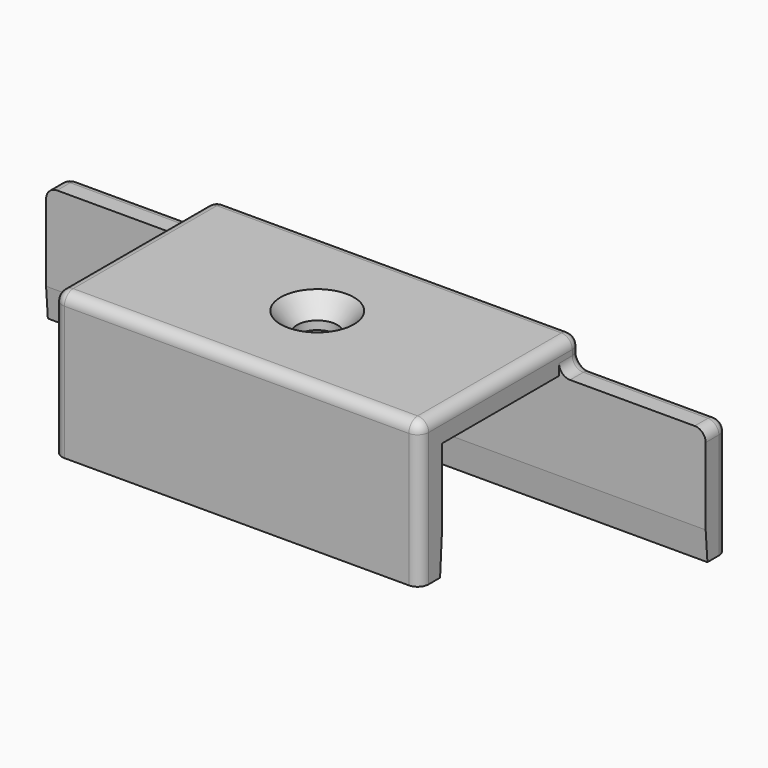
from build123d import *

# Parameters (mm, degrees)
F1_DEPTH       = 31.75
F4_D           = 6.985
F4_DEPTH       = 12.7
F4_CSINK_D     = 12.7
F4_CSINK_ANGLE = 82
F4_TIP         = 2.098505712
F5_SIZE2       = 0.381
F5_SIZE        = 6.35
F2_W           = 4.7625
F2_H           = 20.32
F6_DEPTH       = 25.4
F7_SIZE2       = 5.08
F7_SIZE        = 0.381
F8_R           = 1.905
F9_T1_DEPTH    = 23.1775
F9_T3_DEPTH    = 27.94
F9_S7_W        = 1.905
F9_S7_H        = 1.905
F9_T8_DEPTH    = 1.905
F9_S13_W       = 1.905
F9_S13_H       = 1.905
F9_T14_DEPTH   = 1.905
F9_S19_W       = 1.905
F9_S19_H       = 1.905
F9_T20_DEPTH   = 1.905
F9_S25_W       = 1.905
F9_S25_H       = 1.905
F9_T26_DEPTH   = 1.905


# Not quite as in the source:
# - a fillet or chamfer that OpenCascade refuses, or shapes differently, is made with other operations: its cross-section is extruded or revolved along the edge and cut away or added


with BuildPart() as f1:
    # F0 (on Right) → F1 (new body, symmetric)
    with BuildSketch(Plane.YZ):
        Polygon((-12.7, 0), (-12.7, 20.32), (12.7, 20.32), (12.7, 0), (17.4625, 0), (17.4625, 25.0825), (-17.4625, 25.0825), (-17.4625, 0), align=None)
    extrude(amount=F1_DEPTH, both=True)

    # F4
    with Locations(Plane.XY.offset(25.0825)):
        with Locations((0, 0)):
            CounterSinkHole(F4_D / 2, F4_CSINK_D / 2, depth=F4_DEPTH, counter_sink_angle=F4_CSINK_ANGLE)
            with Locations((0, 0, -(F4_DEPTH + F4_TIP / 2))):  # 118° drill point
                Cone(0, F4_D / 2, F4_TIP, mode=Mode.SUBTRACT)

    # F5
    f5_edges = [f1.edges().sort_by_distance(p)[0] for p in [
        (0, -12.7, 0),
    ]]
    f5_side = f1.faces().sort_by_distance((0, -12.7, 10.16))[0]
    chamfer(f5_edges, length=F5_SIZE, length2=F5_SIZE2, reference=f5_side)

    # F2 (on face) → F6 (join)
    with BuildSketch(Plane(origin=(-31.75, 0, 0), x_dir=(0, -1, 0), z_dir=(-1, 0, 0))):
        with Locations((-15.08125, 10.16)):
            Rectangle(F2_W, F2_H)
    extrude(amount=F6_DEPTH)

    # F7
    f7_edges = [f1.edges().sort_by_distance(p)[0] for p in [
        (-12.7, 12.7, 0),
    ]]
    chamfer(f7_edges, length=F7_SIZE, length2=F7_SIZE2)

    # F8
    f8_edges = [f1.edges().sort_by_distance(p)[0] for p in [
        (-31.75, 0, 25.0825),
        (-31.75, 15.08125, 20.32),
        (-57.15, 15.08125, 20.32),
        (31.75, 0, 25.0825),
        (0, 17.4625, 25.0825),
        (-31.75, 17.4625, 22.70125),
        (-44.45, 17.4625, 20.32),
        (0, -17.4625, 25.0825),
    ]]
    fillet(f8_edges, radius=F8_R)

    # F9: fillet of radius 1.905 on 4 edges, made by hand

    # F9_s2 → F9_t1 (cut)
    with BuildSketch(Plane.XY.offset(-4.7625)):
        with BuildLine():
            ThreePointArc((-55.245, 17.4625), (-56.5920384182, 16.9045384182), (-57.15, 15.5575))
            Line((-57.15, 15.5575), (-57.15, 17.4625))
            Line((-57.15, 17.4625), (-55.245, 17.4625))
        make_face()
    extrude(amount=F9_T1_DEPTH, mode=Mode.SUBTRACT)

    # F9_s4 → F9_t3 (cut)
    with BuildSketch(Plane.XY.offset(-4.7625)):
        with BuildLine():
            ThreePointArc((31.75, 15.5575), (31.1920384182, 16.9045384182), (29.845, 17.4625))
            Line((29.845, 17.4625), (31.75, 17.4625))
            Line((31.75, 17.4625), (31.75, 15.5575))
        make_face()
        with BuildLine():
            ThreePointArc((-29.845, -17.4625), (-31.1920384182, -16.9045384182), (-31.75, -15.5575))
            Line((-31.75, -15.5575), (-31.75, -17.4625))
            Line((-31.75, -17.4625), (-29.845, -17.4625))
        make_face()
        with BuildLine():
            ThreePointArc((31.75, -15.5575), (31.1920384182, -16.9045384182), (29.845, -17.4625))
            Line((29.845, -17.4625), (31.75, -17.4625))
            Line((31.75, -17.4625), (31.75, -15.5575))
        make_face()
    extrude(amount=F9_T3_DEPTH, mode=Mode.SUBTRACT)


with BuildPart() as f9_tool6:
    # F9_s7 → F9_t8 (new body)
    with BuildSketch(Plane.YZ.offset(29.845)):
        with Locations((-16.51, 24.13)):
            Rectangle(F9_S7_W, F9_S7_H)
    extrude(amount=F9_T8_DEPTH)

    # F9_s9 → F9_t10 (revolve, cut)
    with BuildSketch(Plane(origin=(29.845, -15.5575, 23.1775), x_dir=(0, 0.7071067812, -0.7071067812), z_dir=(0, -0.7071067812, -0.7071067812))):
        with BuildLine():
            ThreePointArc((0, -1.905), (1.905, 0), (0, 1.905))
            Line((0, 1.905), (0, -1.905))
        make_face()
    revolve(axis=Axis((29.845, -15.5575, 23.1775), (1, 0, 0)), mode=Mode.SUBTRACT)


with BuildPart() as f1_1:
    add(f1.part)

    # F9_t5: cut F9_tool6
    add(f9_tool6.part, mode=Mode.SUBTRACT)


with BuildPart() as f9_tool12:
    # F9_s13 → F9_t14 (new body)
    with BuildSketch(Plane.XZ.offset(15.5575)):
        with Locations((-30.7975, 24.13)):
            Rectangle(F9_S13_W, F9_S13_H)
    extrude(amount=F9_T14_DEPTH)

    # F9_s15 → F9_t16 (revolve, cut)
    with BuildSketch(Plane(origin=(-29.845, -15.5575, 23.1775), x_dir=(0.7071067812, 0, -0.7071067812), z_dir=(-0.7071067812, 0, -0.7071067812))):
        with BuildLine():
            ThreePointArc((0, -1.905), (1.905, 0), (0, 1.905))
            Line((0, 1.905), (0, -1.905))
        make_face()
    revolve(axis=Axis((-29.845, -15.5575, 23.1775), (0, -1, 0)), mode=Mode.SUBTRACT)


with BuildPart() as f1_2:
    add(f1_1.part)

    # F9_t11: cut F9_tool12
    add(f9_tool12.part, mode=Mode.SUBTRACT)


with BuildPart() as f9_tool18:
    # F9_s19 → F9_t20 (new body)
    with BuildSketch(Plane.YZ.offset(29.845)):
        with Locations((16.51, 24.13)):
            Rectangle(F9_S19_W, F9_S19_H)
    extrude(amount=F9_T20_DEPTH)

    # F9_s21 → F9_t22 (revolve, cut)
    with BuildSketch(Plane(origin=(29.845, 15.5575, 23.1775), x_dir=(0, -0.7071067812, -0.7071067812), z_dir=(0, -0.7071067812, 0.7071067812))):
        with BuildLine():
            ThreePointArc((0, -1.905), (1.905, 0), (0, 1.905))
            Line((0, 1.905), (0, -1.905))
        make_face()
    revolve(axis=Axis((29.845, 15.5575, 23.1775), (1, 0, 0)), mode=Mode.SUBTRACT)


with BuildPart() as f1_3:
    add(f1_2.part)

    # F9_t17: cut F9_tool18
    add(f9_tool18.part, mode=Mode.SUBTRACT)


with BuildPart() as f9_tool24:
    # F9_s25 → F9_t26 (new body)
    with BuildSketch(Plane.XZ.offset(-15.5575)):
        with Locations((-56.1975, 19.3675)):
            Rectangle(F9_S25_W, F9_S25_H)
    extrude(amount=-F9_T26_DEPTH)

    # F9_s27 → F9_t28 (revolve, cut)
    with BuildSketch(Plane(origin=(-55.245, 15.5575, 18.415), x_dir=(0.7071067812, 0, -0.7071067812), z_dir=(0.7071067812, 0, 0.7071067812))):
        with BuildLine():
            ThreePointArc((0, -1.905), (1.905, 0), (0, 1.905))
            Line((0, 1.905), (0, -1.905))
        make_face()
    revolve(axis=Axis((-55.245, 15.5575, 18.415), (0, 1, 0)), mode=Mode.SUBTRACT)


with BuildPart() as f1_4:
    add(f1_3.part)

    # F9_t23: cut F9_tool24
    add(f9_tool24.part, mode=Mode.SUBTRACT)

    # F10: F1 across plane


with BuildPart() as f1_5:
    add(f1_4.part)
    add(f1_4.part.mirror(Plane.YZ))


solid = f1_5.part
